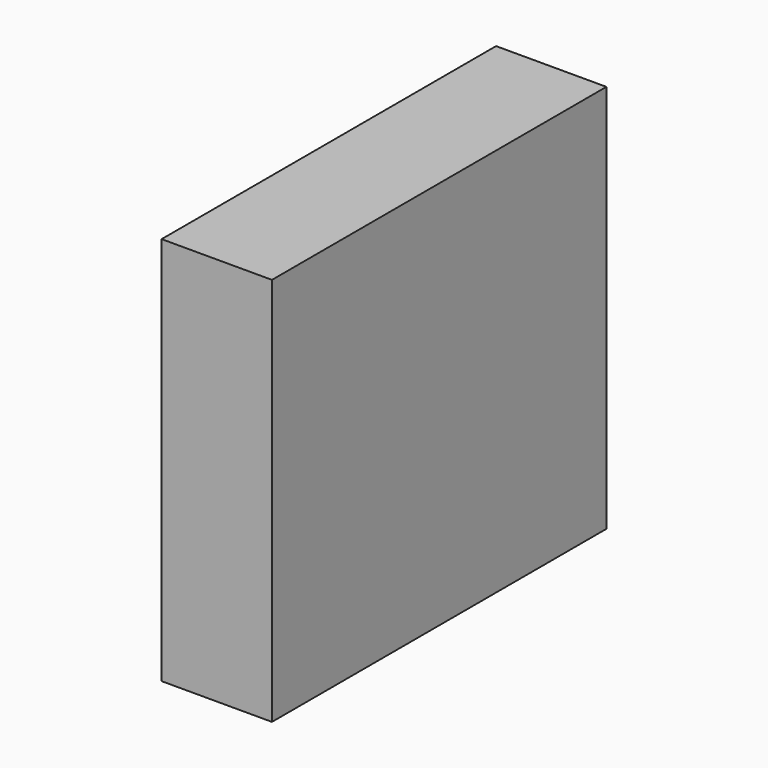
from build123d import *

# Parameters (mm, degrees)
F0_W     = 96.2324663997
F0_H     = 89.5848274231
F1_DEPTH = 25.4


# Not quite as in the source:
# - the program builds the solid bodies; features that only make, move or delete a surface that nothing else refers to are left out


with BuildPart() as f1:
    # F0 (on Right) → F1 (new body)
    with BuildSketch(Plane.YZ):
        Rectangle(F0_W, F0_H)
    extrude(amount=F1_DEPTH)


solid = f1.part
